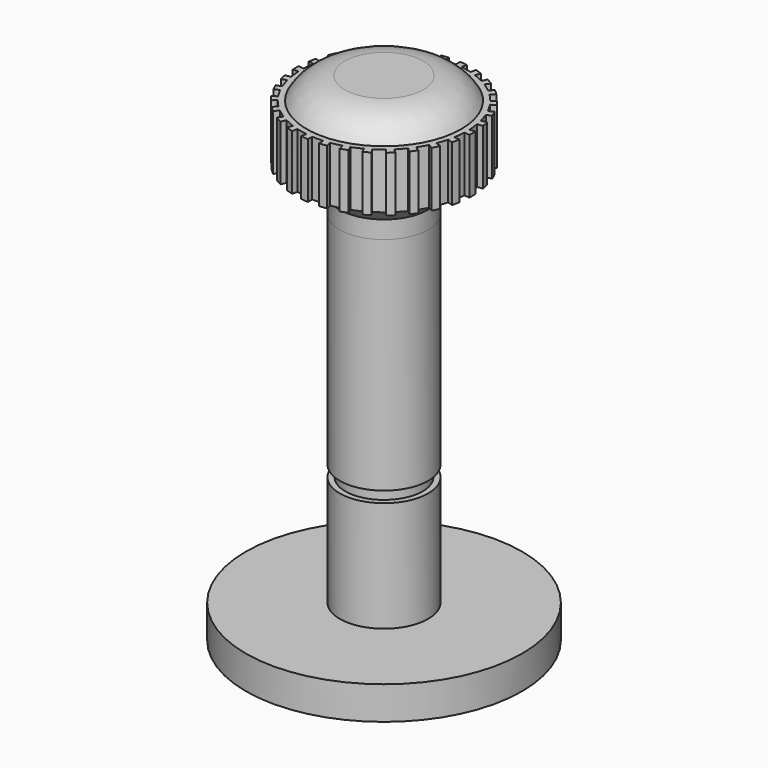
from build123d import *

# Parameters (mm, degrees)
F0_R             = 12.5
F1_DEPTH         = 3
F2_R             = 4
F3_DEPTH         = 10
F4_R             = 3.5
F5_DEPTH         = 1
F6_R             = 4
F7_DEPTH         = 20
F8_R             = 7
F9_DEPTH         = 4
F10_R            = 8
F11_DEPTH        = 5
F12_R            = 7
F13_DEPTH        = 2
F14_S6_R         = 4
F14_T7_DEPTH     = 12
F16_R            = 2
F17_DEPTH        = 10
F19_DEPTH        = 25
F19_COPIES_COUNT = 30


# Not quite as in the source:
# - a fillet or chamfer that OpenCascade refuses, or shapes differently, is made with other operations: its cross-section is extruded or revolved along the edge and cut away or added
# - a pattern or mirror of a feature is missing from the dataset's text; its kind, count and spacing are read off the source's solid


with BuildPart() as f1:
    # F0 (on Top) → F1 (new body)
    with BuildSketch(Plane.XY):
        Circle(F0_R)
    extrude(amount=F1_DEPTH)

    # F2 (on face) → F3 (join)
    with BuildSketch(Plane.XY.offset(3)):
        Circle(F2_R)
    extrude(amount=F3_DEPTH)

    # F4 (on face) → F5 (join)
    with BuildSketch(Plane.XY.offset(13)):
        Circle(F4_R)
    extrude(amount=F5_DEPTH)

    # F6 (on face) → F7 (join)
    with BuildSketch(Plane.XY.offset(14)):
        Circle(F6_R)
    extrude(amount=F7_DEPTH)

    # F8 (on face) → F9 (join)
    with BuildSketch(Plane.XY.offset(34)):
        Circle(F8_R)
    extrude(amount=F9_DEPTH)

    # F10 (on face) → F11 (join)
    with BuildSketch(Plane.XY.offset(38)):
        Circle(F10_R)
    extrude(amount=F11_DEPTH)

    # F12 (on face) → F13 (join)
    with BuildSketch(Plane.XY.offset(43)):
        Circle(F12_R)
    extrude(amount=F13_DEPTH)

    # F14: chamfer of 4 x 5 on 1 edges, made by hand


with BuildPart() as f14_tool2:
    # F14_s3 → F14_t4 (revolve)
    with BuildSketch(Plane.XZ):
        Polygon((7, 38), (2, 34), (7, 34), align=None)
    revolve(axis=Axis((0, 0, 34), (0, 0, 1)))

    split(bisect_by=Plane.XY.offset(38), keep=Keep.BOTTOM)

    # F14_s6 → F14_t7 (cut, symmetric)
    with BuildSketch(Plane.XY.offset(36)):
        Circle(F14_S6_R)
    extrude(amount=F14_T7_DEPTH, both=True, mode=Mode.SUBTRACT)


with BuildPart() as f1_1:
    add(f1.part)

    # F14_t1: cut F14_tool2
    add(f14_tool2.part, mode=Mode.SUBTRACT)

    # F15: fillet of radius 4 on 1 edges, made by hand

    # F15_s1 → F15_t2 (revolve, cut)
    with BuildSketch(Plane.XZ):
        with BuildLine():
            ThreePointArc((7, 43), (5.5358983849, 44.4641016151), (3.5358983849, 45))
            Line((3.5358983849, 45), (7, 45))
            Line((7, 45), (7, 43))
        make_face()
    revolve(axis=Axis((0, 0, 45), (0, 0, 1)), mode=Mode.SUBTRACT)

    # F16 (on face) → F17 (cut)
    with BuildSketch(Plane(origin=(0, 0, 0), x_dir=(1, 0, 0), z_dir=(0, 0, -1))):
        Circle(F16_R)
    extrude(amount=-F17_DEPTH, mode=Mode.SUBTRACT)

    # F18 (on face) → F19 (cut)
    with BuildSketch(Plane.XY.offset(43)):
        with BuildLine():
            ThreePointArc((0.5, 7.9843597113), (0, 8), (-0.5, 7.9843597113))
            Line((-0.5, 7.9843597113), (-0.5, 7.5))
            Line((-0.5, 7.5), (0.5, 7.5))
            Line((0.5, 7.5), (0.5, 7.9843597113))
        make_face()
    f19 = extrude(amount=-F19_DEPTH, mode=Mode.SUBTRACT)

    # F19_copies: F19 ×30 about axis
    f19_copies_axis = Axis((0, 0, 0), (0, 0, 1))
    for i in range(1, F19_COPIES_COUNT):
        add(f19.rotate(f19_copies_axis, i * 360 / F19_COPIES_COUNT), mode=Mode.SUBTRACT)


solid = f1_1.part
